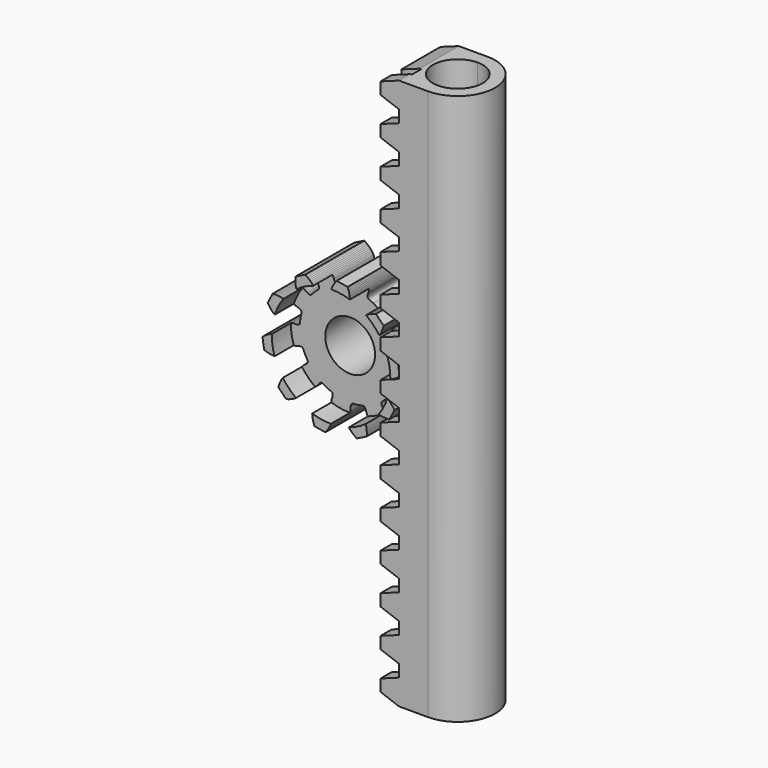
from build123d import *
from build123d import SkipClean  # not in build123d's __all__

# Parameters (mm, degrees)
F1_DEPTH = 19.05
F3_DEPTH = 140.476986
F4_DEPTH = 142.24
F5_DEPTH = 12.7
F6_DEPTH = 18.796
F7_R     = 6.35
F8_DEPTH = 25.4
F2_W     = 4.689856
F2_H     = 3.048
F2_W_2   = 0.390144
F9_DEPTH = 140.476986


with BuildPart() as f1:
    # F0 (on Front) → F1 (new body)
    with BuildSketch(Plane.XZ):
        with BuildLine():
            Line((-37.5894346, 6.493256), (-39.6231013238, 5.7531))
            Line((-39.6231013238, 5.7531), (-30.2295306, 5.7531))
            Line((-30.2295306, 5.7531), (-30.2295306, 73.502774))
            Line((-30.2295306, 73.502774), (-37.5894346, 73.502774))
            Line((-37.5894346, 73.502774), (-42.2792906, 71.79564))
            Line((-42.2792906, 71.79564), (-42.2792906, 68.75145))
            Line((-42.2792906, 68.75145), (-37.5894346, 67.04457))
            Line((-37.5894346, 67.04457), (-37.5894346, 63.930022))
            Line((-37.5894346, 63.930022), (-42.2792906, 62.222888))
            Line((-42.2792906, 62.222888), (-42.2792906, 59.178698))
            Line((-42.2792906, 59.178698), (-37.5894346, 57.471818))
            Line((-37.5894346, 57.471818), (-37.5894346, 54.357016))
            Line((-37.5894346, 54.357016), (-42.2792906, 52.650136))
            Line((-42.2792906, 52.650136), (-42.2792906, 49.605946))
            Line((-42.2792906, 49.605946), (-37.5894346, 47.899066))
            Line((-37.5894346, 47.899066), (-37.5894346, 44.784264))
            Line((-37.5894346, 44.784264), (-42.2792906, 43.077384))
            Line((-42.2792906, 43.077384), (-42.2792906, 40.033194))
            Line((-42.2792906, 40.033194), (-37.5894346, 38.326314))
            Line((-37.5894346, 38.326314), (-37.5894346, 35.211512))
            Line((-37.5894346, 35.211512), (-42.2792906, 33.504632))
            Line((-42.2792906, 33.504632), (-42.2792906, 30.460442))
            Line((-42.2792906, 30.460442), (-37.5894346, 28.753562))
            Line((-37.5894346, 28.753562), (-37.5894346, 25.63876))
            Line((-37.5894346, 25.63876), (-42.2792906, 23.93188))
            Line((-42.2792906, 23.93188), (-42.2792906, 20.88769))
            Line((-42.2792906, 20.88769), (-37.5894346, 19.18081))
            Line((-37.5894346, 19.18081), (-37.5894346, 16.066008))
            Line((-37.5894346, 16.066008), (-42.2792906, 14.359128))
            Line((-42.2792906, 14.359128), (-42.2792906, 13.7205111719))
            ThreePointArc((-42.2792906, 13.7205111719), (-41.5003374209, 12.3003028667), (-40.8778566772, 10.8048840593))
            Line((-40.8778566772, 10.8048840593), (-37.5894346, 9.608058))
            Line((-37.5894346, 9.608058), (-37.5894346, 6.493256))
        make_face()
        with BuildLine():
            ThreePointArc((-40.0091838448, 5.6125846977), (-40.1980996867, 3.3668940627), (-40.7188563132, 1.1742636426))
            Line((-40.7188563132, 1.1742636426), (-37.5894346, 0.035306))
            Line((-37.5894346, 0.035306), (-37.5894346, -3.079496))
            Line((-37.5894346, -3.079496), (-42.2792906, -4.786376))
            Line((-42.2792906, -4.786376), (-42.2792906, -7.830566))
            Line((-42.2792906, -7.830566), (-37.5894346, -9.5377))
            Line((-37.5894346, -9.5377), (-37.5894346, -12.652248))
            Line((-37.5894346, -12.652248), (-42.2792906, -14.359128))
            Line((-42.2792906, -14.359128), (-42.2792906, -17.403318))
            Line((-42.2792906, -17.403318), (-37.5894346, -19.110452))
            Line((-37.5894346, -19.110452), (-37.5894346, -22.225))
            Line((-37.5894346, -22.225), (-42.2792906, -23.93188))
            Line((-42.2792906, -23.93188), (-42.2792906, -26.976324))
            Line((-42.2792906, -26.976324), (-37.5894346, -28.683204))
            Line((-37.5894346, -28.683204), (-37.5894346, -31.797752))
            Line((-37.5894346, -31.797752), (-42.2792906, -33.504632))
            Line((-42.2792906, -33.504632), (-42.2792906, -36.549076))
            Line((-42.2792906, -36.549076), (-37.5894346, -38.255956))
            Line((-37.5894346, -38.255956), (-37.5894346, -41.370504))
            Line((-37.5894346, -41.370504), (-42.2792906, -43.077384))
            Line((-42.2792906, -43.077384), (-42.2792906, -46.121828))
            Line((-42.2792906, -46.121828), (-37.5894346, -47.828708))
            Line((-37.5894346, -47.828708), (-37.5894346, -50.943256))
            Line((-37.5894346, -50.943256), (-42.2792906, -52.650136))
            Line((-42.2792906, -52.650136), (-42.2792906, -55.69458))
            Line((-42.2792906, -55.69458), (-37.5894346, -57.40146))
            Line((-37.5894346, -57.40146), (-37.5894346, -60.516008))
            Line((-37.5894346, -60.516008), (-42.2792906, -62.222888))
            Line((-42.2792906, -62.222888), (-42.2792906, -65.267332))
            Line((-42.2792906, -65.267332), (-37.5894346, -66.974212))
            Line((-37.5894346, -66.974212), (-30.2295306, -66.974212))
            Line((-30.2295306, -66.974212), (-30.2295306, -64.0969))
            Line((-30.2295306, -64.0969), (-30.2295306, 5.7531))
            Line((-30.2295306, 5.7531), (-39.6231013238, 5.7531))
            Line((-39.6231013238, 5.7531), (-40.0091838448, 5.6125846977))
        make_face()
        with BuildLine():
            Line((-42.2792906, 4.786376), (-42.2792906, 1.7442343119))
            Line((-42.2792906, 1.7442343119), (-42.2701137599, 1.7388460755))
            Line((-42.2701137599, 1.7388460755), (-40.7188563132, 1.1742636426))
            ThreePointArc((-40.7188563132, 1.1742636426), (-40.1980996867, 3.3668940627), (-40.0091838448, 5.6125846977))
            Line((-40.0091838448, 5.6125846977), (-42.2792906, 4.786376))
        make_face()
        with BuildLine():
            Line((-42.2792906, 11.314938), (-40.8778566772, 10.8048840593))
            ThreePointArc((-40.8778566772, 10.8048840593), (-41.5003374209, 12.3003028667), (-42.2792906, 13.7205111719))
            Line((-42.2792906, 13.7205111719), (-42.2792906, 11.314938))
        make_face()
    extrude(amount=F1_DEPTH)

    # F2 (on face) → F3 (join, through all)
    with BuildSketch(Plane.XY.offset(73.502774)):
        with BuildLine():
            ThreePointArc((-23.8795306, -9.525), (-25.7394025395, -14.0151280605), (-30.2295306, -15.875))
            Line((-30.2295306, -15.875), (-30.2295306, -19.05))
            ThreePointArc((-30.2295306, -19.05), (-20.7045306, -9.525), (-30.2295306, 0))
            Line((-30.2295306, 0), (-30.2295306, -3.175))
            ThreePointArc((-30.2295306, -3.175), (-25.7394025395, -5.0348719395), (-23.8795306, -9.525))
        make_face()
    extrude(amount=-F3_DEPTH)

    # F2 (on face) → F4 (cut)
    with BuildSketch(Plane.XY.offset(73.502774)):
        with BuildLine():
            Line((-35.8678157116, -12.446), (-30.2295306, -12.446))
            Line((-30.2295306, -12.446), (-30.2295306, -9.525))
            Line((-30.2295306, -9.525), (-30.2295306, -3.175))
            ThreePointArc((-30.2295306, -3.175), (-35.6549729783, -6.2254432116), (-35.8678157116, -12.446))
        make_face()
        with BuildLine():
            Line((-30.2295306, -15.875), (-30.2295306, -12.446))
            Line((-30.2295306, -12.446), (-35.8678157116, -12.446))
            ThreePointArc((-35.8678157116, -12.446), (-33.5290873884, -14.9504423783), (-30.2295306, -15.875))
        make_face()
    with SkipClean():  # cleaning this boolean's faces spoils the solid; the shape is the same uncleaned
        extrude(amount=-F4_DEPTH, mode=Mode.SUBTRACT)

    # F2 (on face) → F9 (cut, through all)
    with BuildSketch(Plane.XY.offset(73.502774)):
        with Locations((-39.9343626, -13.97)):
            Rectangle(F2_W, F2_H)
        with Locations((-37.3943626, -13.97)):
            Rectangle(F2_W_2, F2_H)
    extrude(amount=-F9_DEPTH, mode=Mode.SUBTRACT)


with BuildPart() as f5:
    # F0 (on Front) → F5 (new body)
    with BuildSketch(Plane.XZ):
        with BuildLine():
            Line((-42.7049946, 2.180336), (-42.7217586, 2.410968))
            Line((-42.7217586, 2.410968), (-42.4502326, 3.664458))
            Line((-42.4502326, 3.664458), (-42.3051986, 4.938776))
            Line((-42.3051986, 4.938776), (-42.2150286, 5.151882))
            Line((-42.2150286, 5.151882), (-42.1334946, 5.231638))
            Line((-42.1334946, 5.231638), (-42.0529766, 5.287518))
            Line((-42.0529766, 5.287518), (-41.9734746, 5.330698))
            Line((-41.9734746, 5.330698), (-41.8942266, 5.364734))
            Line((-41.8942266, 5.364734), (-41.7364926, 5.415026))
            Line((-41.7364926, 5.415026), (-41.5792666, 5.447538))
            Line((-41.5792666, 5.447538), (-41.4225486, 5.467096))
            Line((-41.4225486, 5.467096), (-41.2658306, 5.475732))
            Line((-41.2658306, 5.475732), (-40.9534106, 5.467096))
            Line((-40.9534106, 5.467096), (-40.6407366, 5.46354))
            Line((-40.6407366, 5.46354), (-40.3270466, 5.523992))
            Line((-40.3270466, 5.523992), (-40.0131026, 5.614162))
            Line((-40.0131026, 5.614162), (-40.0091561464, 5.6155959101))
            ThreePointArc((-40.0091561464, 5.6155959101), (-40.0086869874, 5.6843472436), (-40.0085306, 5.7531))
            ThreePointArc((-40.0085306, 5.7531), (-40.1905411863, 8.09154481), (-40.7321889245, 10.3736643754))
            Line((-40.7321889245, 10.3736643754), (-40.7364946, 10.373868))
            Line((-40.7364946, 10.373868), (-41.0628846, 10.366756))
            Line((-41.0628846, 10.366756), (-41.3803846, 10.331196))
            Line((-41.3803846, 10.331196), (-41.6778186, 10.23493))
            Line((-41.6778186, 10.23493), (-41.9737286, 10.133838))
            Line((-41.9737286, 10.133838), (-42.1258746, 10.095484))
            Line((-42.1258746, 10.095484), (-42.2813226, 10.067544))
            Line((-42.2813226, 10.067544), (-42.4408346, 10.05205))
            Line((-42.4408346, 10.05205), (-42.6064426, 10.053066))
            Line((-42.6064426, 10.053066), (-42.6922946, 10.06221))
            Line((-42.6922946, 10.06221), (-42.7811946, 10.079482))
            Line((-42.7811946, 10.079482), (-42.8744126, 10.1092))
            Line((-42.8744126, 10.1092), (-42.9762666, 10.161016))
            Line((-42.9762666, 10.161016), (-43.1253646, 10.3378))
            Line((-43.1253646, 10.3378), (-43.6425086, 11.511534))
            Line((-43.6425086, 11.511534), (-44.2742066, 12.62761))
            Line((-44.2742066, 12.62761), (-44.3265306, 12.853162))
            Line((-44.3265306, 12.853162), (-44.3074806, 12.96543))
            Line((-44.3074806, 12.96543), (-44.2752226, 13.05814))
            Line((-44.2752226, 13.05814), (-44.2361066, 13.139674))
            Line((-44.2361066, 13.139674), (-44.1921646, 13.213842))
            Line((-44.1921646, 13.213842), (-44.0941206, 13.347192))
            Line((-44.0941206, 13.347192), (-43.9859166, 13.466064))
            Line((-43.9859166, 13.466064), (-43.8706006, 13.57376))
            Line((-43.8706006, 13.57376), (-43.7489346, 13.67282))
            Line((-43.7489346, 13.67282), (-43.4911246, 13.849604))
            Line((-43.4911246, 13.849604), (-43.2361086, 14.030452))
            Line((-43.2361086, 14.030452), (-43.0176686, 14.263878))
            Line((-43.0176686, 14.263878), (-42.8167546, 14.52118))
            Line((-42.8167546, 14.52118), (-42.8144609172, 14.5245767755))
            ThreePointArc((-42.8144609172, 14.5245767755), (-44.3681141441, 16.3722715085), (-46.1961463252, 17.9490126164))
            Line((-46.1961463252, 17.9490126164), (-46.1997806, 17.946624))
            Line((-46.1997806, 17.946624), (-46.4596226, 17.749012))
            Line((-46.4596226, 17.749012), (-46.6955886, 17.533874))
            Line((-46.6955886, 17.533874), (-46.8797386, 17.28089))
            Line((-46.8797386, 17.28089), (-47.0595706, 17.025366))
            Line((-47.0595706, 17.025366), (-47.1601546, 16.90497))
            Line((-47.1601546, 16.90497), (-47.2693746, 16.790924))
            Line((-47.2693746, 16.790924), (-47.3895166, 16.684498))
            Line((-47.3895166, 16.684498), (-47.5241366, 16.587978))
            Line((-47.5241366, 16.587978), (-47.5988126, 16.545052))
            Line((-47.5988126, 16.545052), (-47.6811086, 16.506952))
            Line((-47.6811086, 16.506952), (-47.7738186, 16.475964))
            Line((-47.7738186, 16.475964), (-47.8865946, 16.45793))
            Line((-47.8865946, 16.45793), (-48.1113846, 16.513302))
            Line((-48.1113846, 16.513302), (-49.2195866, 17.15897))
            Line((-49.2195866, 17.15897), (-50.3864626, 17.690846))
            Line((-50.3864626, 17.690846), (-50.5614686, 17.84223))
            Line((-50.5614686, 17.84223), (-50.6120146, 17.944592))
            Line((-50.6120146, 17.944592), (-50.6404626, 18.038318))
            Line((-50.6404626, 18.038318), (-50.6567186, 18.127218))
            Line((-50.6567186, 18.127218), (-50.6648466, 18.213324))
            Line((-50.6648466, 18.213324), (-50.6638306, 18.378678))
            Line((-50.6638306, 18.378678), (-50.6463046, 18.53819))
            Line((-50.6463046, 18.53819), (-50.6160786, 18.693384))
            Line((-50.6160786, 18.693384), (-50.5762006, 18.845022))
            Line((-50.5762006, 18.845022), (-50.4712986, 19.139408))
            Line((-50.4712986, 19.139408), (-50.3712226, 19.435826))
            Line((-50.3712226, 19.435826), (-50.3318526, 19.752818))
            Line((-50.3318526, 19.752818), (-50.3204226, 20.079208))
            Line((-50.3204226, 20.079208), (-50.3205647885, 20.0832603716))
            ThreePointArc((-50.3205647885, 20.0832603716), (-52.6635401934, 20.6648756207), (-55.0692324438, 20.8660095115))
            Line((-55.0692324438, 20.8660095115), (-55.0707306, 20.862036))
            Line((-55.0707306, 20.862036), (-55.1649646, 20.549362))
            Line((-55.1649646, 20.549362), (-55.2292266, 20.236434))
            Line((-55.2292266, 20.236434), (-55.2294806, 19.92376))
            Line((-55.2294806, 19.92376), (-55.2249086, 19.61134))
            Line((-55.2249086, 19.61134), (-55.2355766, 19.454876))
            Line((-55.2355766, 19.454876), (-55.2569126, 19.298158))
            Line((-55.2569126, 19.298158), (-55.2914566, 19.14144))
            Line((-55.2914566, 19.14144), (-55.3435266, 18.984468))
            Line((-55.3435266, 18.984468), (-55.3788326, 18.905728))
            Line((-55.3788326, 18.905728), (-55.4227746, 18.82648))
            Line((-55.4227746, 18.82648), (-55.4799246, 18.746978))
            Line((-55.4799246, 18.746978), (-55.5604426, 18.666206))
            Line((-55.5604426, 18.666206), (-55.7748186, 18.57883))
            Line((-55.7748186, 18.57883), (-57.0509146, 18.449798))
            Line((-57.0509146, 18.449798), (-58.3077066, 18.19402))
            Line((-58.3077066, 18.19402), (-58.5380846, 18.213832))
            Line((-58.5380846, 18.213832), (-58.6391766, 18.266918))
            Line((-58.6391766, 18.266918), (-58.7171546, 18.325846))
            Line((-58.7171546, 18.325846), (-58.7826866, 18.38833))
            Line((-58.7826866, 18.38833), (-58.8398366, 18.4531))
            Line((-58.8398366, 18.4531), (-58.9363566, 18.58772))
            Line((-58.9363566, 18.58772), (-59.0158586, 18.727166))
            Line((-59.0158586, 18.727166), (-59.0826606, 18.870168))
            Line((-59.0826606, 18.870168), (-59.1393026, 19.016472))
            Line((-59.1393026, 19.016472), (-59.2276946, 19.316446))
            Line((-59.2276946, 19.316446), (-59.3209126, 19.614896))
            Line((-59.3209126, 19.614896), (-59.4753446, 19.89455))
            Line((-59.4753446, 19.89455), (-59.6579706, 20.16506))
            Line((-59.6579706, 20.16506), (-59.6605550865, 20.1683705736))
            ThreePointArc((-59.6605550865, 20.1683705736), (-61.8979124478, 19.2617423468), (-63.9623690599, 18.0104383867))
            Line((-63.9623690599, 18.0104383867), (-63.9612386, 18.006314))
            Line((-63.9612386, 18.006314), (-63.8535426, 17.698212))
            Line((-63.8535426, 17.698212), (-63.7219706, 17.407128))
            Line((-63.7219706, 17.407128), (-63.5383286, 17.15389))
            Line((-63.5383286, 17.15389), (-63.3506226, 16.903954))
            Line((-63.3506226, 16.903954), (-63.2673106, 16.771112))
            Line((-63.2673106, 16.771112), (-63.1926346, 16.63192))
            Line((-63.1926346, 16.63192), (-63.1286266, 16.484854))
            Line((-63.1286266, 16.484854), (-63.0783346, 16.326866))
            Line((-63.0783346, 16.326866), (-63.0605546, 16.242538))
            Line((-63.0605546, 16.242538), (-63.0496326, 16.152622))
            Line((-63.0496326, 16.152622), (-63.0488706, 16.054832))
            Line((-63.0488706, 16.054832), (-63.0669046, 15.942056))
            Line((-63.0669046, 15.942056), (-63.1888246, 15.74546))
            Line((-63.1888246, 15.74546), (-64.1451346, 14.891004))
            Line((-64.1451346, 14.891004), (-65.0117826, 13.945362))
            Line((-65.0117826, 13.945362), (-65.2099026, 13.825728))
            Line((-65.2099026, 13.825728), (-65.3226786, 13.809472))
            Line((-65.3226786, 13.809472), (-65.4207226, 13.81125))
            Line((-65.4207226, 13.81125), (-65.5103846, 13.823442))
            Line((-65.5103846, 13.823442), (-65.5944586, 13.842238))
            Line((-65.5944586, 13.842238), (-65.7516846, 13.894308))
            Line((-65.7516846, 13.894308), (-65.8979886, 13.960348))
            Line((-65.8979886, 13.960348), (-66.0361646, 14.036802))
            Line((-66.0361646, 14.036802), (-66.1679906, 14.121638))
            Line((-66.1679906, 14.121638), (-66.4156406, 14.312392))
            Line((-66.4156406, 14.312392), (-66.6665926, 14.499082))
            Line((-66.6665926, 14.499082), (-66.9558986, 14.634718))
            Line((-66.9558986, 14.634718), (-67.2627306, 14.746224))
            Line((-67.2627306, 14.746224), (-67.266728965, 14.7473718257))
            ThreePointArc((-67.266728965, 14.7473718257), (-68.5439005812, 12.6988003309), (-69.478593619, 10.4730057691))
            Line((-69.478593619, 10.4730057691), (-69.4753246, 10.470388))
            Line((-69.4753246, 10.470388), (-69.2071006, 10.284206))
            Line((-69.2071006, 10.284206), (-68.9294786, 10.126218))
            Line((-68.9294786, 10.126218), (-68.6320446, 10.029444))
            Line((-68.6320446, 10.029444), (-68.3333406, 9.937242))
            Line((-68.3333406, 9.937242), (-68.1877986, 9.878822))
            Line((-68.1877986, 9.878822), (-68.0455586, 9.810242))
            Line((-68.0455586, 9.810242), (-67.9071286, 9.728962))
            Line((-67.9071286, 9.728962), (-67.7740326, 9.630664))
            Line((-67.7740326, 9.630664), (-67.7097706, 9.572752))
            Line((-67.7097706, 9.572752), (-67.6483026, 9.506458))
            Line((-67.6483026, 9.506458), (-67.5901366, 9.427718))
            Line((-67.5901366, 9.427718), (-67.5383206, 9.326118))
            Line((-67.5383206, 9.326118), (-67.5215566, 9.095232))
            Line((-67.5215566, 9.095232), (-67.7928286, 7.841742))
            Line((-67.7928286, 7.841742), (-67.9381166, 6.567424))
            Line((-67.9381166, 6.567424), (-68.0280326, 6.354318))
            Line((-68.0280326, 6.354318), (-68.1098206, 6.274562))
            Line((-68.1098206, 6.274562), (-68.1900846, 6.218682))
            Line((-68.1900846, 6.218682), (-68.2698406, 6.175756))
            Line((-68.2698406, 6.175756), (-68.3490886, 6.141466))
            Line((-68.3490886, 6.141466), (-68.5068226, 6.091174))
            Line((-68.5068226, 6.091174), (-68.6640486, 6.058662))
            Line((-68.6640486, 6.058662), (-68.8207666, 6.039358))
            Line((-68.8207666, 6.039358), (-68.9772306, 6.030468))
            Line((-68.9772306, 6.030468), (-69.2899046, 6.039104))
            Line((-69.2899046, 6.039104), (-69.6023246, 6.042914))
            Line((-69.6023246, 6.042914), (-69.9162686, 5.982462))
            Line((-69.9162686, 5.982462), (-70.2299586, 5.892292))
            Line((-70.2299586, 5.892292), (-70.2339027327, 5.8908589331))
            ThreePointArc((-70.2339027327, 5.8908589331), (-70.0630419578, 3.4828561045), (-69.5109501969, 1.1327782942))
            Line((-69.5109501969, 1.1327782942), (-69.5068206, 1.132586))
            Line((-69.5068206, 1.132586), (-69.1804306, 1.139698))
            Line((-69.1804306, 1.139698), (-68.8626766, 1.175004))
            Line((-68.8626766, 1.175004), (-68.5652426, 1.271524))
            Line((-68.5652426, 1.271524), (-68.2695866, 1.372616))
            Line((-68.2695866, 1.372616), (-68.1174406, 1.410716))
            Line((-68.1174406, 1.410716), (-67.9619926, 1.43891))
            Line((-67.9619926, 1.43891), (-67.8022266, 1.454404))
            Line((-67.8022266, 1.454404), (-67.6366186, 1.453388))
            Line((-67.6366186, 1.453388), (-67.5507666, 1.444244))
            Line((-67.5507666, 1.444244), (-67.4618666, 1.426718))
            Line((-67.4618666, 1.426718), (-67.3686486, 1.397254))
            Line((-67.3686486, 1.397254), (-67.2670486, 1.345438))
            Line((-67.2670486, 1.345438), (-67.1176966, 1.1684))
            Line((-67.1176966, 1.1684), (-66.6005526, -0.00508))
            Line((-66.6005526, -0.00508), (-65.9691086, -1.12141))
            Line((-65.9691086, -1.12141), (-65.9165306, -1.346708))
            Line((-65.9165306, -1.346708), (-65.9358346, -1.45923))
            Line((-65.9358346, -1.45923), (-65.9678386, -1.551686))
            Line((-65.9678386, -1.551686), (-66.0069546, -1.63322))
            Line((-66.0069546, -1.63322), (-66.0511506, -1.707642))
            Line((-66.0511506, -1.707642), (-66.1491946, -1.840992))
            Line((-66.1491946, -1.840992), (-66.2571446, -1.95961))
            Line((-66.2571446, -1.95961), (-66.3727146, -2.06756))
            Line((-66.3727146, -2.06756), (-66.4941266, -2.16662))
            Line((-66.4941266, -2.16662), (-66.7519366, -2.34315))
            Line((-66.7519366, -2.34315), (-67.0072066, -2.523998))
            Line((-67.0072066, -2.523998), (-67.2253926, -2.757424))
            Line((-67.2253926, -2.757424), (-67.4263066, -3.014726))
            Line((-67.4263066, -3.014726), (-67.4286872297, -3.0182547808))
            ThreePointArc((-67.4286872297, -3.0182547808), (-65.8750513507, -4.8659658942), (-64.0470335444, -6.4427257691))
            Line((-64.0470335444, -6.4427257691), (-64.0435346, -6.440424))
            Line((-64.0435346, -6.440424), (-63.7836926, -6.242812))
            Line((-63.7836926, -6.242812), (-63.5474726, -6.02742))
            Line((-63.5474726, -6.02742), (-63.3635766, -5.77469))
            Line((-63.3635766, -5.77469), (-63.1834906, -5.518912))
            Line((-63.1834906, -5.518912), (-63.0829066, -5.39877))
            Line((-63.0829066, -5.39877), (-62.9736866, -5.284724))
            Line((-62.9736866, -5.284724), (-62.8535446, -5.178044))
            Line((-62.8535446, -5.178044), (-62.7191786, -5.081778))
            Line((-62.7191786, -5.081778), (-62.6442486, -5.038598))
            Line((-62.6442486, -5.038598), (-62.5622066, -5.000498))
            Line((-62.5622066, -5.000498), (-62.4692426, -4.96951))
            Line((-62.4692426, -4.96951), (-62.3564666, -4.95173))
            Line((-62.3564666, -4.95173), (-62.1319306, -5.007102))
            Line((-62.1319306, -5.007102), (-61.0237286, -5.652516))
            Line((-61.0237286, -5.652516), (-59.8565986, -6.184392))
            Line((-59.8565986, -6.184392), (-59.6815926, -6.335776))
            Line((-59.6815926, -6.335776), (-59.6310466, -6.438138))
            Line((-59.6310466, -6.438138), (-59.6028526, -6.531864))
            Line((-59.6028526, -6.531864), (-59.5865966, -6.621018))
            Line((-59.5865966, -6.621018), (-59.5784686, -6.70687))
            Line((-59.5784686, -6.70687), (-59.5794846, -6.872478))
            Line((-59.5794846, -6.872478), (-59.5970106, -7.03199))
            Line((-59.5970106, -7.03199), (-59.6269826, -7.187184))
            Line((-59.6269826, -7.187184), (-59.6671146, -7.338568))
            Line((-59.6671146, -7.338568), (-59.7717626, -7.633208))
            Line((-59.7717626, -7.633208), (-59.8720926, -7.929372))
            Line((-59.8720926, -7.929372), (-59.9114626, -8.246618))
            Line((-59.9114626, -8.246618), (-59.9226386, -8.572754))
            Line((-59.9226386, -8.572754), (-59.9224908326, -8.5770622407))
            ThreePointArc((-59.9224908326, -8.5770622407), (-57.5795203011, -9.158675737), (-55.1738332098, -9.3598094961))
            Line((-55.1738332098, -9.3598094961), (-55.1723306, -9.355836))
            Line((-55.1723306, -9.355836), (-55.0783506, -9.043162))
            Line((-55.0783506, -9.043162), (-55.0138346, -8.730234))
            Line((-55.0138346, -8.730234), (-55.0135806, -8.41756))
            Line((-55.0135806, -8.41756), (-55.0184066, -8.104886))
            Line((-55.0184066, -8.104886), (-55.0077386, -7.948422))
            Line((-55.0077386, -7.948422), (-54.9861486, -7.791958))
            Line((-54.9861486, -7.791958), (-54.9516046, -7.63524))
            Line((-54.9516046, -7.63524), (-54.8995346, -7.478014))
            Line((-54.8995346, -7.478014), (-54.8642286, -7.399274))
            Line((-54.8642286, -7.399274), (-54.8202866, -7.32028))
            Line((-54.8202866, -7.32028), (-54.7633906, -7.240524))
            Line((-54.7633906, -7.240524), (-54.6826186, -7.160006))
            Line((-54.6826186, -7.160006), (-54.4682426, -7.07263))
            Line((-54.4682426, -7.07263), (-53.1924006, -6.943344))
            Line((-53.1924006, -6.943344), (-51.9356086, -6.68782))
            Line((-51.9356086, -6.68782), (-51.7049766, -6.707378))
            Line((-51.7049766, -6.707378), (-51.6038846, -6.760464))
            Line((-51.6038846, -6.760464), (-51.5259066, -6.819646))
            Line((-51.5259066, -6.819646), (-51.4603746, -6.88213))
            Line((-51.4603746, -6.88213), (-51.4034786, -6.9469))
            Line((-51.4034786, -6.9469), (-51.3069586, -7.08152))
            Line((-51.3069586, -7.08152), (-51.2274566, -7.220712))
            Line((-51.2274566, -7.220712), (-51.1604006, -7.363968))
            Line((-51.1604006, -7.363968), (-51.1037586, -7.510018))
            Line((-51.1037586, -7.510018), (-51.0153666, -7.809992))
            Line((-51.0153666, -7.809992), (-50.9224026, -8.108442))
            Line((-50.9224026, -8.108442), (-50.7677166, -8.388096))
            Line((-50.7677166, -8.388096), (-50.5850906, -8.65886))
            Line((-50.5850906, -8.65886), (-50.5825066772, -8.6621707511))
            ThreePointArc((-50.5825066772, -8.6621707511), (-48.3451501056, -7.7555430257), (-46.2806941169, -6.5042398125))
            Line((-46.2806941169, -6.5042398125), (-46.2818226, -6.500114))
            Line((-46.2818226, -6.500114), (-46.3895186, -6.191758))
            Line((-46.3895186, -6.191758), (-46.5213446, -5.900674))
            Line((-46.5213446, -5.900674), (-46.7049866, -5.64769))
            Line((-46.7049866, -5.64769), (-46.8924386, -5.3975))
            Line((-46.8924386, -5.3975), (-46.9757506, -5.264658))
            Line((-46.9757506, -5.264658), (-47.0504266, -5.125466))
            Line((-47.0504266, -5.125466), (-47.1146886, -4.9784))
            Line((-47.1146886, -4.9784), (-47.1647266, -4.820666))
            Line((-47.1647266, -4.820666), (-47.1825066, -4.736084))
            Line((-47.1825066, -4.736084), (-47.1934286, -4.646422))
            Line((-47.1934286, -4.646422), (-47.1941906, -4.548378))
            Line((-47.1941906, -4.548378), (-47.1764106, -4.435602))
            Line((-47.1764106, -4.435602), (-47.0542366, -4.239006))
            Line((-47.0542366, -4.239006), (-46.0979266, -3.38455))
            Line((-46.0979266, -3.38455), (-45.2315326, -2.438908))
            Line((-45.2315326, -2.438908), (-45.0334126, -2.319528))
            Line((-45.0334126, -2.319528), (-44.9203826, -2.303018))
            Line((-44.9203826, -2.303018), (-44.8225926, -2.30505))
            Line((-44.8225926, -2.30505), (-44.7329306, -2.316988))
            Line((-44.7329306, -2.316988), (-44.6486026, -2.335784))
            Line((-44.6486026, -2.335784), (-44.4913766, -2.388108))
            Line((-44.4913766, -2.388108), (-44.3450726, -2.453894))
            Line((-44.3450726, -2.453894), (-44.2068966, -2.530348))
            Line((-44.2068966, -2.530348), (-44.0750706, -2.615438))
            Line((-44.0750706, -2.615438), (-43.8274206, -2.806192))
            Line((-43.8274206, -2.806192), (-43.5767226, -2.992882))
            Line((-43.5767226, -2.992882), (-43.2871626, -3.128264))
            Line((-43.2871626, -3.128264), (-42.9803306, -3.23977))
            Line((-42.9803306, -3.23977), (-42.9761791238, -3.240965072))
            ThreePointArc((-42.9761791238, -3.240965072), (-41.6990534876, -1.1923932991), (-40.7644023284, 1.0333927217))
            Line((-40.7644023284, 1.0333927217), (-40.7677366, 1.036066))
            Line((-40.7677366, 1.036066), (-41.0359606, 1.221994))
            Line((-41.0359606, 1.221994), (-41.3138366, 1.379982))
            Line((-41.3138366, 1.379982), (-41.6110166, 1.47701))
            Line((-41.6110166, 1.47701), (-41.9099746, 1.568958))
            Line((-41.9099746, 1.568958), (-42.0552626, 1.627632))
            Line((-42.0552626, 1.627632), (-42.1975026, 1.696212))
            Line((-42.1975026, 1.696212), (-42.2701137599, 1.7388460755))
            Line((-42.2701137599, 1.7388460755), (-42.2792906, 1.742186))
            Line((-42.2792906, 1.742186), (-42.2792906, 1.7442343119))
            Line((-42.2792906, 1.7442343119), (-42.3359326, 1.777492))
            Line((-42.3359326, 1.777492), (-42.4692826, 1.875536))
            Line((-42.4692826, 1.875536), (-42.5332906, 1.933448))
            Line((-42.5332906, 1.933448), (-42.5950126, 1.999742))
            Line((-42.5950126, 1.999742), (-42.6531786, 2.078736))
            Line((-42.6531786, 2.078736), (-42.7049946, 2.180336))
        make_face()
        with BuildLine():
            ThreePointArc((-46.1961463252, 17.9490126164), (-44.3681141441, 16.3722715085), (-42.8144609172, 14.5245767755))
            Line((-42.8144609172, 14.5245767755), (-42.6303186, 14.797278))
            Line((-42.6303186, 14.797278), (-42.4568366, 15.089886))
            Line((-42.4568366, 15.089886), (-42.2960546, 15.39748))
            Line((-42.2960546, 15.39748), (-42.1474646, 15.718536))
            Line((-42.1474646, 15.718536), (-42.0108126, 16.052292))
            Line((-42.0108126, 16.052292), (-41.8860986, 16.397986))
            Line((-41.8860986, 16.397986), (-41.7735766, 16.754856))
            Line((-41.7735766, 16.754856), (-41.6973766, 17.029684))
            Line((-41.6973766, 17.029684), (-43.6773066, 19.03476))
            Line((-43.6773066, 19.03476), (-43.9528966, 18.961862))
            Line((-43.9528966, 18.961862), (-44.3112906, 18.853658))
            Line((-44.3112906, 18.853658), (-44.6585086, 18.733516))
            Line((-44.6585086, 18.733516), (-44.9940426, 18.601182))
            Line((-44.9940426, 18.601182), (-45.3168766, 18.456402))
            Line((-45.3168766, 18.456402), (-45.6265026, 18.29943))
            Line((-45.6265026, 18.29943), (-45.9211426, 18.129758))
            Line((-45.9211426, 18.129758), (-46.1961463252, 17.9490126164))
        make_face()
        with BuildLine():
            ThreePointArc((-40.7321889245, 10.3736643754), (-40.1905411863, 8.09154481), (-40.0085306, 5.7531))
            Line((-40.0085306, 5.7531), (-39.6417201593, 5.7531))
            Line((-39.6417201593, 5.7531), (-39.3877546, 5.862828))
            Line((-39.3877546, 5.862828), (-39.0768586, 6.016752))
            Line((-39.0768586, 6.016752), (-38.7677406, 6.189218))
            Line((-38.7677406, 6.189218), (-38.4611626, 6.378956))
            Line((-38.4611626, 6.378956), (-38.1571246, 6.585458))
            Line((-38.1571246, 6.585458), (-37.8561346, 6.807962))
            Line((-37.8561346, 6.807962), (-37.6328686, 6.985508))
            Line((-37.6328686, 6.985508), (-38.0562866, 9.77138))
            Line((-38.0562866, 9.77138), (-38.3222246, 9.874504))
            Line((-38.3222246, 9.874504), (-38.6755386, 9.997694))
            Line((-38.6755386, 9.997694), (-39.0270746, 10.104628))
            Line((-39.0270746, 10.104628), (-39.3763246, 10.194544))
            Line((-39.3763246, 10.194544), (-39.7225266, 10.267442))
            Line((-39.7225266, 10.267442), (-40.0651726, 10.322306))
            Line((-40.0651726, 10.322306), (-40.4035006, 10.35812))
            Line((-40.4035006, 10.35812), (-40.7321889245, 10.3736643754))
        make_face()
        with BuildLine():
            Line((-40.5076406, 0.827532), (-40.7644023284, 1.0333927217))
            ThreePointArc((-40.7644023284, 1.0333927217), (-41.6990534876, -1.1923932991), (-42.9761791238, -3.240965072))
            Line((-42.9761791238, -3.240965072), (-42.6600366, -3.331972))
            Line((-42.6600366, -3.331972), (-42.3280586, -3.406394))
            Line((-42.3280586, -3.406394), (-41.9861746, -3.464306))
            Line((-41.9861746, -3.464306), (-41.6348926, -3.506724))
            Line((-41.6348926, -3.506724), (-41.2752286, -3.533394))
            Line((-41.2752286, -3.533394), (-40.9079446, -3.545078))
            Line((-40.9079446, -3.545078), (-40.5335486, -3.541776))
            Line((-40.5335486, -3.541776), (-40.2485606, -3.529584))
            Line((-40.2485606, -3.529584), (-38.9536686, -1.026922))
            Line((-38.9536686, -1.026922), (-39.1081006, -0.787146))
            Line((-39.1081006, -0.787146), (-39.3217146, -0.479552))
            Line((-39.3217146, -0.479552), (-39.5432026, -0.18669))
            Line((-39.5432026, -0.18669), (-39.7728186, 0.09144))
            Line((-39.7728186, 0.09144), (-40.0103086, 0.354076))
            Line((-40.0103086, 0.354076), (-40.2551646, 0.599694))
            Line((-40.2551646, 0.599694), (-40.5076406, 0.827532))
        make_face()
        with BuildLine():
            Line((-46.1939386, -6.821424), (-46.2806941169, -6.5042398125))
            ThreePointArc((-46.2806941169, -6.5042398125), (-48.3451501056, -7.7555430257), (-50.5825066772, -8.6621707511))
            Line((-50.5825066772, -8.6621707511), (-50.3801126, -8.921496))
            Line((-50.3801126, -8.921496), (-50.1553226, -9.176766))
            Line((-50.1553226, -9.176766), (-49.9127526, -9.424924))
            Line((-49.9127526, -9.424924), (-49.6534186, -9.665462))
            Line((-49.6534186, -9.665462), (-49.3780826, -9.898634))
            Line((-49.3780826, -9.898634), (-49.0877606, -10.123932))
            Line((-49.0877606, -10.123932), (-48.7829606, -10.341102))
            Line((-48.7829606, -10.341102), (-48.5452166, -10.498836))
            Line((-48.5452166, -10.498836), (-46.0265526, -9.235186))
            Line((-46.0265526, -9.235186), (-46.0108046, -8.950452))
            Line((-46.0108046, -8.950452), (-46.0026766, -8.57631))
            Line((-46.0026766, -8.57631), (-46.0097886, -8.208772))
            Line((-46.0097886, -8.208772), (-46.0321406, -7.848854))
            Line((-46.0321406, -7.848854), (-46.0697326, -7.497064))
            Line((-46.0697326, -7.497064), (-46.1235806, -7.154418))
            Line((-46.1235806, -7.154418), (-46.1939386, -6.821424))
        make_face()
        with BuildLine():
            Line((-55.2901866, -9.667494), (-55.1738332098, -9.3598094961))
            ThreePointArc((-55.1738332098, -9.3598094961), (-57.5795203011, -9.158675737), (-59.9224908326, -8.5770622407))
            Line((-59.9224908326, -8.5770622407), (-59.9112086, -8.906002))
            Line((-59.9112086, -8.906002), (-59.8794586, -9.244584))
            Line((-59.8794586, -9.244584), (-59.8289126, -9.587738))
            Line((-59.8289126, -9.587738), (-59.7605866, -9.934956))
            Line((-59.7605866, -9.934956), (-59.6747346, -10.285222))
            Line((-59.6747346, -10.285222), (-59.5723726, -10.638282))
            Line((-59.5723726, -10.638282), (-59.4535006, -10.99312))
            Line((-59.4535006, -10.99312), (-59.3539326, -11.260328))
            Line((-59.3539326, -11.260328), (-56.5736486, -11.718544))
            Line((-56.5736486, -11.718544), (-56.3933086, -11.497564))
            Line((-56.3933086, -11.497564), (-56.1669946, -11.199622))
            Line((-56.1669946, -11.199622), (-55.9566826, -10.898124))
            Line((-55.9566826, -10.898124), (-55.7631346, -10.593832))
            Line((-55.7631346, -10.593832), (-55.5868586, -10.287))
            Line((-55.5868586, -10.287), (-55.4288706, -9.978136))
            Line((-55.4288706, -9.978136), (-55.2901866, -9.667494))
        make_face()
        with BuildLine():
            Line((-64.3219186, -6.623558), (-64.0470335444, -6.4427257691))
            ThreePointArc((-64.0470335444, -6.4427257691), (-65.8750513507, -4.8659658942), (-67.4286872297, -3.0182547808))
            Line((-67.4286872297, -3.0182547808), (-67.6127426, -3.291078))
            Line((-67.6127426, -3.291078), (-67.7862246, -3.583686))
            Line((-67.7862246, -3.583686), (-67.9470066, -3.891026))
            Line((-67.9470066, -3.891026), (-68.0958506, -4.212082))
            Line((-68.0958506, -4.212082), (-68.2325026, -4.545838))
            Line((-68.2325026, -4.545838), (-68.3569626, -4.891532))
            Line((-68.3569626, -4.891532), (-68.4694846, -5.248656))
            Line((-68.4694846, -5.248656), (-68.5459386, -5.523484))
            Line((-68.5459386, -5.523484), (-66.5660086, -7.528306))
            Line((-66.5660086, -7.528306), (-66.2901646, -7.455408))
            Line((-66.2901646, -7.455408), (-65.9317706, -7.347458))
            Line((-65.9317706, -7.347458), (-65.5845526, -7.227316))
            Line((-65.5845526, -7.227316), (-65.2490186, -7.094728))
            Line((-65.2490186, -7.094728), (-64.9261846, -6.950202))
            Line((-64.9261846, -6.950202), (-64.6168126, -6.79323))
            Line((-64.6168126, -6.79323), (-64.3219186, -6.623558))
        make_face()
        with BuildLine():
            Line((-69.8395606, 1.14808), (-69.5109501969, 1.1327782942))
            ThreePointArc((-69.5109501969, 1.1327782942), (-70.0630419578, 3.4828561045), (-70.2339027327, 5.8908589331))
            Line((-70.2339027327, 5.8908589331), (-70.5431406, 5.7785))
            Line((-70.5431406, 5.7785), (-70.8555606, 5.643626))
            Line((-70.8555606, 5.643626), (-71.1664566, 5.489448))
            Line((-71.1664566, 5.489448), (-71.4753206, 5.317236))
            Line((-71.4753206, 5.317236), (-71.7821526, 5.127498))
            Line((-71.7821526, 5.127498), (-72.0861906, 4.920996))
            Line((-72.0861906, 4.920996), (-72.3869266, 4.698238))
            Line((-72.3869266, 4.698238), (-72.6101926, 4.520946))
            Line((-72.6101926, 4.520946), (-72.1870286, 1.735074))
            Line((-72.1870286, 1.735074), (-71.9210906, 1.63195))
            Line((-71.9210906, 1.63195), (-71.5675226, 1.50876))
            Line((-71.5675226, 1.50876), (-71.2159866, 1.401826))
            Line((-71.2159866, 1.401826), (-70.8667366, 1.311656))
            Line((-70.8667366, 1.311656), (-70.5205346, 1.239012))
            Line((-70.5205346, 1.239012), (-70.1778886, 1.184148))
            Line((-70.1778886, 1.184148), (-69.8395606, 1.14808))
        make_face()
        with BuildLine():
            Line((-69.7354206, 10.678668), (-69.478593619, 10.4730057691))
            ThreePointArc((-69.478593619, 10.4730057691), (-68.5439005812, 12.6988003309), (-67.266728965, 14.7473718257))
            Line((-67.266728965, 14.7473718257), (-67.5830246, 14.838172))
            Line((-67.5830246, 14.838172), (-67.9150026, 14.912848))
            Line((-67.9150026, 14.912848), (-68.2571406, 14.97076))
            Line((-68.2571406, 14.97076), (-68.6084226, 15.012924))
            Line((-68.6084226, 15.012924), (-68.9680866, 15.039848))
            Line((-68.9680866, 15.039848), (-69.3353706, 15.051278))
            Line((-69.3353706, 15.051278), (-69.7095126, 15.047976))
            Line((-69.7095126, 15.047976), (-69.9945006, 15.035784))
            Line((-69.9945006, 15.035784), (-71.2896466, 12.533122))
            Line((-71.2896466, 12.533122), (-71.1349606, 12.293346))
            Line((-71.1349606, 12.293346), (-70.9216006, 11.986006))
            Line((-70.9216006, 11.986006), (-70.6998586, 11.69289))
            Line((-70.6998586, 11.69289), (-70.4702426, 11.41476))
            Line((-70.4702426, 11.41476), (-70.2330066, 11.152378))
            Line((-70.2330066, 11.152378), (-69.9878966, 10.906506))
            Line((-69.9878966, 10.906506), (-69.7354206, 10.678668))
        make_face()
        with BuildLine():
            ThreePointArc((-63.9623690599, 18.0104383867), (-61.8979124478, 19.2617423468), (-59.6605550865, 20.1683705736))
            Line((-59.6605550865, 20.1683705736), (-59.8632026, 20.42795))
            Line((-59.8632026, 20.42795), (-60.0877386, 20.68322))
            Line((-60.0877386, 20.68322), (-60.3305626, 20.931124))
            Line((-60.3305626, 20.931124), (-60.5898966, 21.171916))
            Line((-60.5898966, 21.171916), (-60.8649786, 21.404834))
            Line((-60.8649786, 21.404834), (-61.1553006, 21.630132))
            Line((-61.1553006, 21.630132), (-61.4601006, 21.847556))
            Line((-61.4601006, 21.847556), (-61.6978446, 22.005036))
            Line((-61.6978446, 22.005036), (-64.2165086, 20.74164))
            Line((-64.2165086, 20.74164), (-64.2325106, 20.456906))
            Line((-64.2325106, 20.456906), (-64.2403846, 20.08251))
            Line((-64.2403846, 20.08251), (-64.2335266, 19.715226))
            Line((-64.2335266, 19.715226), (-64.2111746, 19.355308))
            Line((-64.2111746, 19.355308), (-64.1733286, 19.003518))
            Line((-64.1733286, 19.003518), (-64.1197346, 18.660618))
            Line((-64.1197346, 18.660618), (-64.0493766, 18.327878))
            Line((-64.0493766, 18.327878), (-63.9623690599, 18.0104383867))
        make_face()
        with BuildLine():
            ThreePointArc((-55.0692324438, 20.8660095115), (-52.6635401934, 20.6648756207), (-50.3205647885, 20.0832603716))
            Line((-50.3205647885, 20.0832603716), (-50.3321066, 20.412202))
            Line((-50.3321066, 20.412202), (-50.3636026, 20.750784))
            Line((-50.3636026, 20.750784), (-50.4141486, 21.094192))
            Line((-50.4141486, 21.094192), (-50.4827286, 21.44141))
            Line((-50.4827286, 21.44141), (-50.5683266, 21.791676))
            Line((-50.5683266, 21.791676), (-50.6706886, 22.144482))
            Line((-50.6706886, 22.144482), (-50.7895606, 22.499574))
            Line((-50.7895606, 22.499574), (-50.8893826, 22.766782))
            Line((-50.8893826, 22.766782), (-53.6696666, 23.224998))
            Line((-53.6696666, 23.224998), (-53.8497526, 23.004018))
            Line((-53.8497526, 23.004018), (-54.0763206, 22.705822))
            Line((-54.0763206, 22.705822), (-54.2866326, 22.404578))
            Line((-54.2866326, 22.404578), (-54.4801806, 22.100286))
            Line((-54.4801806, 22.100286), (-54.6562026, 21.793454))
            Line((-54.6562026, 21.793454), (-54.8144446, 21.48459))
            Line((-54.8144446, 21.48459), (-54.9531286, 21.173948))
            Line((-54.9531286, 21.173948), (-55.0692324438, 20.8660095115))
        make_face()
        with BuildLine():
            ThreePointArc((-40.0085306, 5.7531), (-40.0086869874, 5.6843472436), (-40.0091561464, 5.6155959101))
            Line((-40.0091561464, 5.6155959101), (-39.6999206, 5.727954))
            Line((-39.6999206, 5.727954), (-39.6417201593, 5.7531))
            Line((-39.6417201593, 5.7531), (-40.0085306, 5.7531))
        make_face()
    extrude(amount=F5_DEPTH)

    # F0 (on Front) → F6 (join)
    with BuildSketch(Plane.XZ):
        with BuildLine():
            ThreePointArc((-46.1961463252, 17.9490126164), (-44.3681141441, 16.3722715085), (-42.8144609172, 14.5245767755))
            Line((-42.8144609172, 14.5245767755), (-42.6303186, 14.797278))
            Line((-42.6303186, 14.797278), (-42.4568366, 15.089886))
            Line((-42.4568366, 15.089886), (-42.2960546, 15.39748))
            Line((-42.2960546, 15.39748), (-42.1474646, 15.718536))
            Line((-42.1474646, 15.718536), (-42.0108126, 16.052292))
            Line((-42.0108126, 16.052292), (-41.8860986, 16.397986))
            Line((-41.8860986, 16.397986), (-41.7735766, 16.754856))
            Line((-41.7735766, 16.754856), (-41.6973766, 17.029684))
            Line((-41.6973766, 17.029684), (-43.6773066, 19.03476))
            Line((-43.6773066, 19.03476), (-43.9528966, 18.961862))
            Line((-43.9528966, 18.961862), (-44.3112906, 18.853658))
            Line((-44.3112906, 18.853658), (-44.6585086, 18.733516))
            Line((-44.6585086, 18.733516), (-44.9940426, 18.601182))
            Line((-44.9940426, 18.601182), (-45.3168766, 18.456402))
            Line((-45.3168766, 18.456402), (-45.6265026, 18.29943))
            Line((-45.6265026, 18.29943), (-45.9211426, 18.129758))
            Line((-45.9211426, 18.129758), (-46.1961463252, 17.9490126164))
        make_face()
        with BuildLine():
            ThreePointArc((-55.0692324438, 20.8660095115), (-52.6635401934, 20.6648756207), (-50.3205647885, 20.0832603716))
            Line((-50.3205647885, 20.0832603716), (-50.3321066, 20.412202))
            Line((-50.3321066, 20.412202), (-50.3636026, 20.750784))
            Line((-50.3636026, 20.750784), (-50.4141486, 21.094192))
            Line((-50.4141486, 21.094192), (-50.4827286, 21.44141))
            Line((-50.4827286, 21.44141), (-50.5683266, 21.791676))
            Line((-50.5683266, 21.791676), (-50.6706886, 22.144482))
            Line((-50.6706886, 22.144482), (-50.7895606, 22.499574))
            Line((-50.7895606, 22.499574), (-50.8893826, 22.766782))
            Line((-50.8893826, 22.766782), (-53.6696666, 23.224998))
            Line((-53.6696666, 23.224998), (-53.8497526, 23.004018))
            Line((-53.8497526, 23.004018), (-54.0763206, 22.705822))
            Line((-54.0763206, 22.705822), (-54.2866326, 22.404578))
            Line((-54.2866326, 22.404578), (-54.4801806, 22.100286))
            Line((-54.4801806, 22.100286), (-54.6562026, 21.793454))
            Line((-54.6562026, 21.793454), (-54.8144446, 21.48459))
            Line((-54.8144446, 21.48459), (-54.9531286, 21.173948))
            Line((-54.9531286, 21.173948), (-55.0692324438, 20.8660095115))
        make_face()
        with BuildLine():
            ThreePointArc((-63.9623690599, 18.0104383867), (-61.8979124478, 19.2617423468), (-59.6605550865, 20.1683705736))
            Line((-59.6605550865, 20.1683705736), (-59.8632026, 20.42795))
            Line((-59.8632026, 20.42795), (-60.0877386, 20.68322))
            Line((-60.0877386, 20.68322), (-60.3305626, 20.931124))
            Line((-60.3305626, 20.931124), (-60.5898966, 21.171916))
            Line((-60.5898966, 21.171916), (-60.8649786, 21.404834))
            Line((-60.8649786, 21.404834), (-61.1553006, 21.630132))
            Line((-61.1553006, 21.630132), (-61.4601006, 21.847556))
            Line((-61.4601006, 21.847556), (-61.6978446, 22.005036))
            Line((-61.6978446, 22.005036), (-64.2165086, 20.74164))
            Line((-64.2165086, 20.74164), (-64.2325106, 20.456906))
            Line((-64.2325106, 20.456906), (-64.2403846, 20.08251))
            Line((-64.2403846, 20.08251), (-64.2335266, 19.715226))
            Line((-64.2335266, 19.715226), (-64.2111746, 19.355308))
            Line((-64.2111746, 19.355308), (-64.1733286, 19.003518))
            Line((-64.1733286, 19.003518), (-64.1197346, 18.660618))
            Line((-64.1197346, 18.660618), (-64.0493766, 18.327878))
            Line((-64.0493766, 18.327878), (-63.9623690599, 18.0104383867))
        make_face()
        with BuildLine():
            Line((-69.7354206, 10.678668), (-69.478593619, 10.4730057691))
            ThreePointArc((-69.478593619, 10.4730057691), (-68.5439005812, 12.6988003309), (-67.266728965, 14.7473718257))
            Line((-67.266728965, 14.7473718257), (-67.5830246, 14.838172))
            Line((-67.5830246, 14.838172), (-67.9150026, 14.912848))
            Line((-67.9150026, 14.912848), (-68.2571406, 14.97076))
            Line((-68.2571406, 14.97076), (-68.6084226, 15.012924))
            Line((-68.6084226, 15.012924), (-68.9680866, 15.039848))
            Line((-68.9680866, 15.039848), (-69.3353706, 15.051278))
            Line((-69.3353706, 15.051278), (-69.7095126, 15.047976))
            Line((-69.7095126, 15.047976), (-69.9945006, 15.035784))
            Line((-69.9945006, 15.035784), (-71.2896466, 12.533122))
            Line((-71.2896466, 12.533122), (-71.1349606, 12.293346))
            Line((-71.1349606, 12.293346), (-70.9216006, 11.986006))
            Line((-70.9216006, 11.986006), (-70.6998586, 11.69289))
            Line((-70.6998586, 11.69289), (-70.4702426, 11.41476))
            Line((-70.4702426, 11.41476), (-70.2330066, 11.152378))
            Line((-70.2330066, 11.152378), (-69.9878966, 10.906506))
            Line((-69.9878966, 10.906506), (-69.7354206, 10.678668))
        make_face()
        with BuildLine():
            Line((-69.8395606, 1.14808), (-69.5109501969, 1.1327782942))
            ThreePointArc((-69.5109501969, 1.1327782942), (-70.0630419578, 3.4828561045), (-70.2339027327, 5.8908589331))
            Line((-70.2339027327, 5.8908589331), (-70.5431406, 5.7785))
            Line((-70.5431406, 5.7785), (-70.8555606, 5.643626))
            Line((-70.8555606, 5.643626), (-71.1664566, 5.489448))
            Line((-71.1664566, 5.489448), (-71.4753206, 5.317236))
            Line((-71.4753206, 5.317236), (-71.7821526, 5.127498))
            Line((-71.7821526, 5.127498), (-72.0861906, 4.920996))
            Line((-72.0861906, 4.920996), (-72.3869266, 4.698238))
            Line((-72.3869266, 4.698238), (-72.6101926, 4.520946))
            Line((-72.6101926, 4.520946), (-72.1870286, 1.735074))
            Line((-72.1870286, 1.735074), (-71.9210906, 1.63195))
            Line((-71.9210906, 1.63195), (-71.5675226, 1.50876))
            Line((-71.5675226, 1.50876), (-71.2159866, 1.401826))
            Line((-71.2159866, 1.401826), (-70.8667366, 1.311656))
            Line((-70.8667366, 1.311656), (-70.5205346, 1.239012))
            Line((-70.5205346, 1.239012), (-70.1778886, 1.184148))
            Line((-70.1778886, 1.184148), (-69.8395606, 1.14808))
        make_face()
        with BuildLine():
            ThreePointArc((-40.7321889245, 10.3736643754), (-40.1905411863, 8.09154481), (-40.0085306, 5.7531))
            Line((-40.0085306, 5.7531), (-39.6417201593, 5.7531))
            Line((-39.6417201593, 5.7531), (-39.3877546, 5.862828))
            Line((-39.3877546, 5.862828), (-39.0768586, 6.016752))
            Line((-39.0768586, 6.016752), (-38.7677406, 6.189218))
            Line((-38.7677406, 6.189218), (-38.4611626, 6.378956))
            Line((-38.4611626, 6.378956), (-38.1571246, 6.585458))
            Line((-38.1571246, 6.585458), (-37.8561346, 6.807962))
            Line((-37.8561346, 6.807962), (-37.6328686, 6.985508))
            Line((-37.6328686, 6.985508), (-38.0562866, 9.77138))
            Line((-38.0562866, 9.77138), (-38.3222246, 9.874504))
            Line((-38.3222246, 9.874504), (-38.6755386, 9.997694))
            Line((-38.6755386, 9.997694), (-39.0270746, 10.104628))
            Line((-39.0270746, 10.104628), (-39.3763246, 10.194544))
            Line((-39.3763246, 10.194544), (-39.7225266, 10.267442))
            Line((-39.7225266, 10.267442), (-40.0651726, 10.322306))
            Line((-40.0651726, 10.322306), (-40.4035006, 10.35812))
            Line((-40.4035006, 10.35812), (-40.7321889245, 10.3736643754))
        make_face()
        with BuildLine():
            Line((-40.5076406, 0.827532), (-40.7644023284, 1.0333927217))
            ThreePointArc((-40.7644023284, 1.0333927217), (-41.6990534876, -1.1923932991), (-42.9761791238, -3.240965072))
            Line((-42.9761791238, -3.240965072), (-42.6600366, -3.331972))
            Line((-42.6600366, -3.331972), (-42.3280586, -3.406394))
            Line((-42.3280586, -3.406394), (-41.9861746, -3.464306))
            Line((-41.9861746, -3.464306), (-41.6348926, -3.506724))
            Line((-41.6348926, -3.506724), (-41.2752286, -3.533394))
            Line((-41.2752286, -3.533394), (-40.9079446, -3.545078))
            Line((-40.9079446, -3.545078), (-40.5335486, -3.541776))
            Line((-40.5335486, -3.541776), (-40.2485606, -3.529584))
            Line((-40.2485606, -3.529584), (-38.9536686, -1.026922))
            Line((-38.9536686, -1.026922), (-39.1081006, -0.787146))
            Line((-39.1081006, -0.787146), (-39.3217146, -0.479552))
            Line((-39.3217146, -0.479552), (-39.5432026, -0.18669))
            Line((-39.5432026, -0.18669), (-39.7728186, 0.09144))
            Line((-39.7728186, 0.09144), (-40.0103086, 0.354076))
            Line((-40.0103086, 0.354076), (-40.2551646, 0.599694))
            Line((-40.2551646, 0.599694), (-40.5076406, 0.827532))
        make_face()
        with BuildLine():
            Line((-46.1939386, -6.821424), (-46.2806941169, -6.5042398125))
            ThreePointArc((-46.2806941169, -6.5042398125), (-48.3451501056, -7.7555430257), (-50.5825066772, -8.6621707511))
            Line((-50.5825066772, -8.6621707511), (-50.3801126, -8.921496))
            Line((-50.3801126, -8.921496), (-50.1553226, -9.176766))
            Line((-50.1553226, -9.176766), (-49.9127526, -9.424924))
            Line((-49.9127526, -9.424924), (-49.6534186, -9.665462))
            Line((-49.6534186, -9.665462), (-49.3780826, -9.898634))
            Line((-49.3780826, -9.898634), (-49.0877606, -10.123932))
            Line((-49.0877606, -10.123932), (-48.7829606, -10.341102))
            Line((-48.7829606, -10.341102), (-48.5452166, -10.498836))
            Line((-48.5452166, -10.498836), (-46.0265526, -9.235186))
            Line((-46.0265526, -9.235186), (-46.0108046, -8.950452))
            Line((-46.0108046, -8.950452), (-46.0026766, -8.57631))
            Line((-46.0026766, -8.57631), (-46.0097886, -8.208772))
            Line((-46.0097886, -8.208772), (-46.0321406, -7.848854))
            Line((-46.0321406, -7.848854), (-46.0697326, -7.497064))
            Line((-46.0697326, -7.497064), (-46.1235806, -7.154418))
            Line((-46.1235806, -7.154418), (-46.1939386, -6.821424))
        make_face()
        with BuildLine():
            Line((-55.2901866, -9.667494), (-55.1738332098, -9.3598094961))
            ThreePointArc((-55.1738332098, -9.3598094961), (-57.5795203011, -9.158675737), (-59.9224908326, -8.5770622407))
            Line((-59.9224908326, -8.5770622407), (-59.9112086, -8.906002))
            Line((-59.9112086, -8.906002), (-59.8794586, -9.244584))
            Line((-59.8794586, -9.244584), (-59.8289126, -9.587738))
            Line((-59.8289126, -9.587738), (-59.7605866, -9.934956))
            Line((-59.7605866, -9.934956), (-59.6747346, -10.285222))
            Line((-59.6747346, -10.285222), (-59.5723726, -10.638282))
            Line((-59.5723726, -10.638282), (-59.4535006, -10.99312))
            Line((-59.4535006, -10.99312), (-59.3539326, -11.260328))
            Line((-59.3539326, -11.260328), (-56.5736486, -11.718544))
            Line((-56.5736486, -11.718544), (-56.3933086, -11.497564))
            Line((-56.3933086, -11.497564), (-56.1669946, -11.199622))
            Line((-56.1669946, -11.199622), (-55.9566826, -10.898124))
            Line((-55.9566826, -10.898124), (-55.7631346, -10.593832))
            Line((-55.7631346, -10.593832), (-55.5868586, -10.287))
            Line((-55.5868586, -10.287), (-55.4288706, -9.978136))
            Line((-55.4288706, -9.978136), (-55.2901866, -9.667494))
        make_face()
        with BuildLine():
            Line((-64.3219186, -6.623558), (-64.0470335444, -6.4427257691))
            ThreePointArc((-64.0470335444, -6.4427257691), (-65.8750513507, -4.8659658942), (-67.4286872297, -3.0182547808))
            Line((-67.4286872297, -3.0182547808), (-67.6127426, -3.291078))
            Line((-67.6127426, -3.291078), (-67.7862246, -3.583686))
            Line((-67.7862246, -3.583686), (-67.9470066, -3.891026))
            Line((-67.9470066, -3.891026), (-68.0958506, -4.212082))
            Line((-68.0958506, -4.212082), (-68.2325026, -4.545838))
            Line((-68.2325026, -4.545838), (-68.3569626, -4.891532))
            Line((-68.3569626, -4.891532), (-68.4694846, -5.248656))
            Line((-68.4694846, -5.248656), (-68.5459386, -5.523484))
            Line((-68.5459386, -5.523484), (-66.5660086, -7.528306))
            Line((-66.5660086, -7.528306), (-66.2901646, -7.455408))
            Line((-66.2901646, -7.455408), (-65.9317706, -7.347458))
            Line((-65.9317706, -7.347458), (-65.5845526, -7.227316))
            Line((-65.5845526, -7.227316), (-65.2490186, -7.094728))
            Line((-65.2490186, -7.094728), (-64.9261846, -6.950202))
            Line((-64.9261846, -6.950202), (-64.6168126, -6.79323))
            Line((-64.6168126, -6.79323), (-64.3219186, -6.623558))
        make_face()
    extrude(amount=F6_DEPTH)

    # F7 (on face) → F8 (cut)
    with BuildSketch(Plane.XZ):
        with Locations((-55.1215306, 5.7531)):
            Circle(F7_R)
    extrude(amount=F8_DEPTH, mode=Mode.SUBTRACT)


solid = Compound([f1.part, f5.part])
